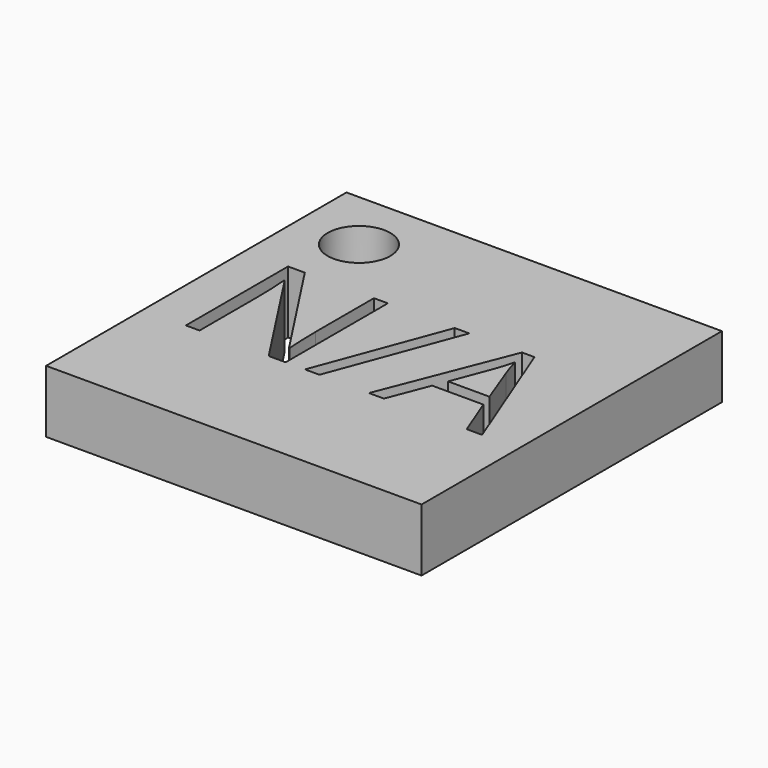
from build123d import *

# Parameters (mm, degrees)
F0_W         = 30
F0_H         = 30
F0_R         = 2.5
F1_DEPTH     = 5
F2_TEXT_SIZE = 14.295532646
F3_DEPTH     = 5.001


# Not quite as in the source:
# - Text() gives the source's letters only with a copy of the font that has no kerning and outlines rounded to 1/6400 em; it was checked with that copy


with BuildPart() as f1:
    # F0 (on Top) → F1 (new body)
    with BuildSketch(Plane.XY):
        with Locations((15, 15)):
            Rectangle(F0_W, F0_H)
        with Locations((5, 25)):
            Circle(F0_R, mode=Mode.SUBTRACT)
    extrude(amount=F1_DEPTH)

    # F2 (on face) → F3 (cut, through all)
    with BuildSketch(Plane.XY.offset(5)):
        with Locations((2, 9.7072164948)):
            Text('N/A', F2_TEXT_SIZE, font='Open Sans', text_align=(TextAlign.LEFT, TextAlign.BOTTOM))
    extrude(amount=-F3_DEPTH, mode=Mode.SUBTRACT)


solid = f1.part
